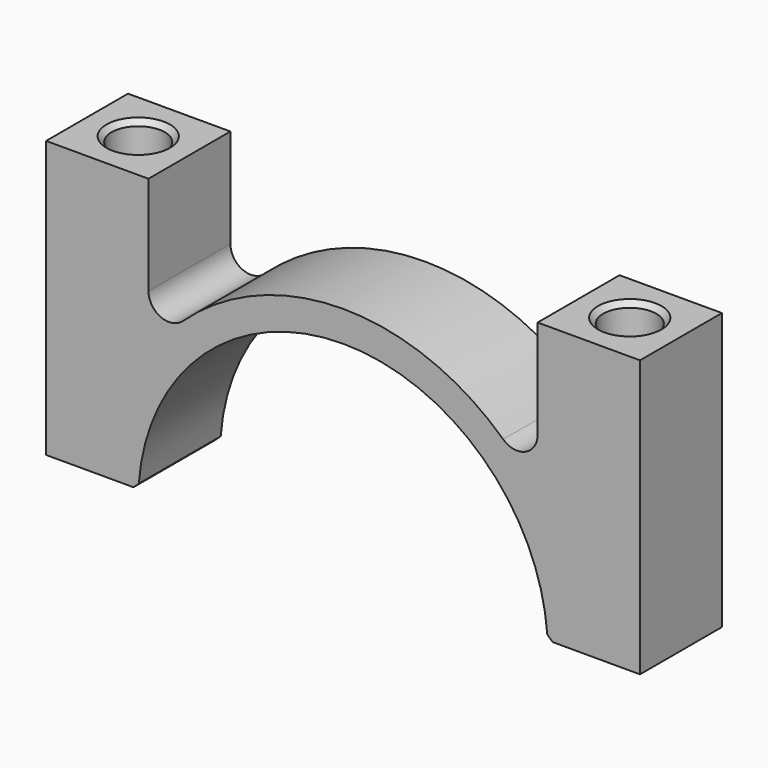
from build123d import *

# Parameters (mm, degrees)
F1_DEPTH    = 5
F2_T1_DEPTH = 6.2718359258
F2_T3_DEPTH = 6.2718359258
F3_R        = 2.6
F4_DEPTH    = 27.001
F5_SIZE     = 0.5


# Not quite as in the source:
# - a fillet or chamfer that OpenCascade refuses, or shapes differently, is made with other operations: its cross-section is extruded or revolved along the edge and cut away or added
# - a pattern or mirror of a feature is missing from the dataset's text; its kind, count and spacing are read off the source's solid


with BuildPart() as f1:
    # F0 (on Front) → F1 (new body, symmetric)
    with BuildSketch(Plane.XZ):
        with BuildLine():
            ThreePointArc((0, 20), (13.7840487521, 14.4913767462), (19.9749843554, 1))
            Line((19.9749843554, 1), (29, 1))
            Line((29, 1), (29, 28))
            Line((29, 28), (19, 28))
            Line((19, 28), (19, 18.3303027798))
            ThreePointArc((19, 18.3303027798), (17.8, 16.4972725018), (15.64, 16.8638785574))
            ThreePointArc((15.64, 16.8638785574), (8.4003212194, 21.4110859933), (0, 23))
            ThreePointArc((0, 23), (-8.4003212194, 21.4110859933), (-15.64, 16.8638785574))
            ThreePointArc((-15.64, 16.8638785574), (-17.8, 16.4972725018), (-19, 18.3303027798))
            Line((-19, 18.3303027798), (-19, 28))
            Line((-19, 28), (-29, 28))
            Line((-29, 28), (-29, 1))
            Line((-29, 1), (-19.9749843554, 1))
            ThreePointArc((-19.9749843554, 1), (-13.7840487521, 14.4913767462), (0, 20))
        make_face()
    extrude(amount=F1_DEPTH, both=True)

    # F2: chamfer of 0.5 on 4 edges, made by hand

    # F2_s2 → F2_t1 (cut)
    with BuildSketch(Plane.XZ.offset(-6.2718359258)):
        with BuildLine():
            Line((19.9300167465, 1.500192138), (20.4835367376, 0.9863935992))
            Line((20.4835367376, 0.9863935992), (20.4835367376, 0.9763935992))
            ThreePointArc((20.4835367376, 0.9763935992), (20.2292605465, 0.99), (19.9749843554, 0.99))
            Line((19.9749843554, 0.99), (19.9649968633, 0.9995))
            ThreePointArc((19.9649968633, 0.9995), (19.9508800221, 1.249994537), (19.920044409, 1.4994488451))
            Line((19.920044409, 1.4994488451), (19.9300167465, 1.500192138))
        make_face()
        with BuildLine():
            Line((-19.9300167465, 1.500192138), (-20.4835367376, 0.9863935992))
            Line((-20.4835367376, 0.9863935992), (-20.4835367376, 0.9763935992))
            ThreePointArc((-20.4835367376, 0.9763935992), (-20.2292605465, 0.99), (-19.9749843554, 0.99))
            Line((-19.9749843554, 0.99), (-19.9649968633, 0.9995))
            ThreePointArc((-19.9649968633, 0.9995), (-19.9508800221, 1.249994537), (-19.920044409, 1.4994488451))
            Line((-19.920044409, 1.4994488451), (-19.9300167465, 1.500192138))
        make_face()
    extrude(amount=F2_T1_DEPTH, mode=Mode.SUBTRACT)

    # F2_s4 → F2_t3 (cut)
    with BuildSketch(Plane.XZ):
        with BuildLine():
            Line((19.9300167465, 1.500192138), (20.4835367376, 0.9863935992))
            Line((20.4835367376, 0.9863935992), (20.4835367376, 0.9763935992))
            ThreePointArc((20.4835367376, 0.9763935992), (20.2292605465, 0.99), (19.9749843554, 0.99))
            Line((19.9749843554, 0.99), (19.9649968633, 0.9995))
            ThreePointArc((19.9649968633, 0.9995), (19.9508800221, 1.249994537), (19.920044409, 1.4994488451))
            Line((19.920044409, 1.4994488451), (19.9300167465, 1.500192138))
        make_face()
        with BuildLine():
            Line((-19.9300167465, 1.500192138), (-20.4835367376, 0.9863935992))
            Line((-20.4835367376, 0.9863935992), (-20.4835367376, 0.9763935992))
            ThreePointArc((-20.4835367376, 0.9763935992), (-20.2292605465, 0.99), (-19.9749843554, 0.99))
            Line((-19.9749843554, 0.99), (-19.9649968633, 0.9995))
            ThreePointArc((-19.9649968633, 0.9995), (-19.9508800221, 1.249994537), (-19.920044409, 1.4994488451))
            Line((-19.920044409, 1.4994488451), (-19.9300167465, 1.500192138))
        make_face()
    extrude(amount=F2_T3_DEPTH, mode=Mode.SUBTRACT)

    # F3 (on face) → F4 (cut, through all)
    with BuildSketch(Plane.XY.offset(28)):
        with Locations((24, 0)):
            Circle(F3_R)
    f4 = extrude(amount=-F4_DEPTH, mode=Mode.SUBTRACT)

    # F4_copies: F4 across plane
    add(f4.mirror(Plane(origin=(0, 0, 0), x_dir=(0, 0, -1), z_dir=(-1, 0, 0))), mode=Mode.SUBTRACT)

    # F5
    f5_edges = [f1.edges().sort_by_distance(p)[0] for p in [
        (24, 2.6, 28),
        (24, -2.6, 28),
        (24, 2.6, 1),
        (-24, 2.6, 1),
        (-24, 2.6, 28),
        (24, -2.6, 1),
        (-24, -2.6, 1),
        (-24, -2.6, 28),
    ]]
    chamfer(f5_edges, length=F5_SIZE)


solid = f1.part
